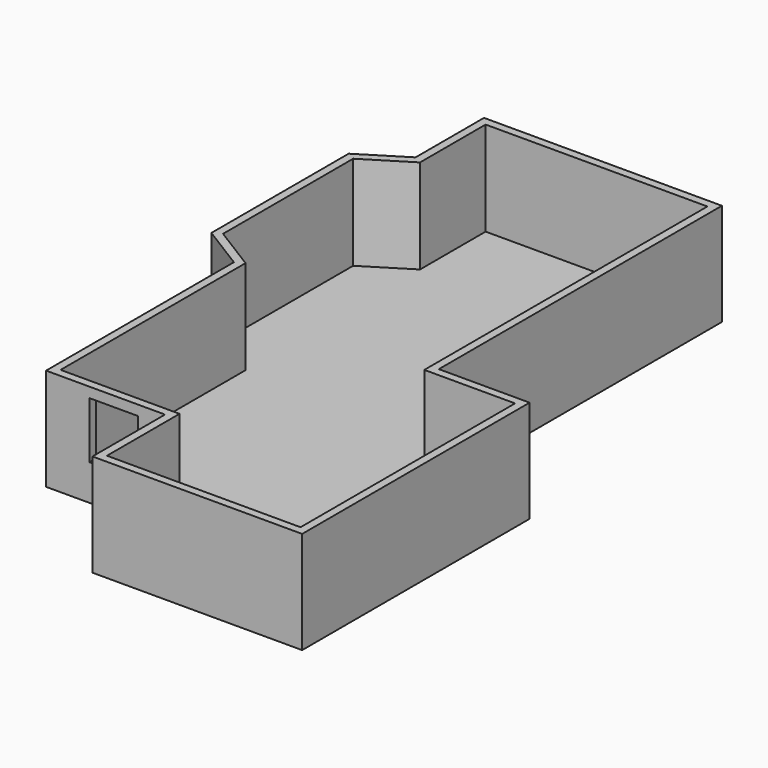
from build123d import *

# Parameters (mm, degrees)
F1_DEPTH = 2578.1
F2_T     = -203.2
F3_W     = 1219.2
F3_H     = 1422.4
F5_DEPTH = 203.2


# Not quite as in the source:
# - a feature of the source that left no trace in its solid (it failed there, or was rolled back) is left out


with BuildPart() as f1:
    # F0 (on Top) → F1 (new body)
    with BuildSketch(Plane.XY):
        Polygon((-2286, 16078.2), (-8280.4, 16078.2), (-8280.4, 13922.375), (-9406.501324312, 13223.08125), (-9406.501324312, 8900.31875), (-8280.4, 8201.025), (-8280.4, 2286), (-5283.2, 2286), (-5283.2, 0), (0, 0), (0, 7162.8), (-2286, 7162.8), align=None)
    extrude(amount=F1_DEPTH)

    # F2
    f2_openings = [f1.faces().sort_by_distance(p)[0] for p in [
        (-4762.628229, 7961.579676, 2578.1),
    ]]
    offset(amount=F2_T, openings=f2_openings, kind=Kind.INTERSECTION)

    # F3 (on face) → F5 (cut, through all)
    with BuildSketch(Plane(origin=(0, 2489.2, 0), x_dir=(-1, 0, 0), z_dir=(0, 1, 0))):
        with Locations((6578.6, 1612.9)):
            Rectangle(F3_W, F3_H)
    extrude(amount=-F5_DEPTH, mode=Mode.SUBTRACT)


solid = f1.part
